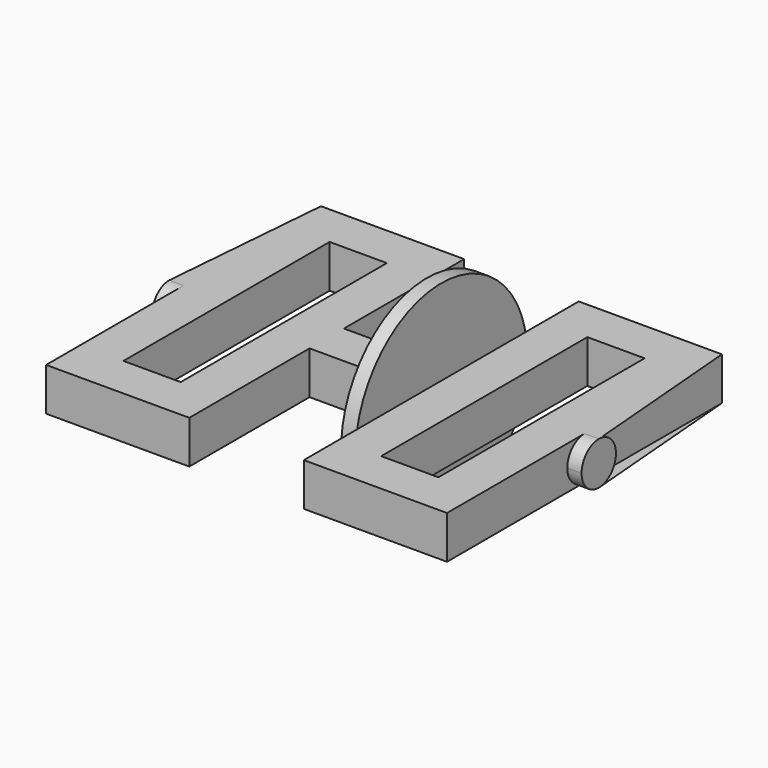
from build123d import *

# Parameters (mm, degrees)
F0_W     = 10
F0_H     = 30
F0_W_2   = 40
F0_H_2   = 180
F0_W_3   = 80
F1_DEPTH = 15
F2_R     = 15
F3_R     = 14.99999
F5_START = 30
F4_R     = 75
F5_DEPTH = 10


# Not quite as in the source:
# - a fillet or chamfer is up to 0.001 mm smaller than in the source, because OpenCascade refuses the exact size


with BuildPart() as f1:
    # F0 (on Top) → F1 (new body, symmetric)
    with BuildSketch(Plane.XY):
        with Locations((-145, 0)):
            Rectangle(F0_W, F0_H)
        Polygon((-140, 120), (-140, 15), (-140, -15), (-140, -120), (-40, -120), (-40, -15), (-40, 15), (-40, 120), align=None)
        with Locations((-90, 0)):
            Rectangle(F0_W_2, F0_H_2, mode=Mode.SUBTRACT)
        Rectangle(F0_W_3, F0_H)
        Polygon((40, 120), (40, 15), (40, -15), (40, -120), (140, -120), (140, -15), (140, 15), (140, 120), align=None)
        with Locations((90, 0)):
            Rectangle(F0_W_2, F0_H_2, mode=Mode.SUBTRACT)
        with Locations((145, 0)):
            Rectangle(F0_W, F0_H)
    extrude(amount=F1_DEPTH, both=True)

    # F2
    f2_edges = [f1.edges().sort_by_distance(p)[0] for p in [
        (-145, -15, 15),
    ]]
    fillet(f2_edges, radius=F2_R)

    # F3 (radius 15 in the source; OpenCascade refuses exactly that, so slightly less here)
    f3_edges = [f1.edges().sort_by_distance(p)[0] for p in [
        (-145, -15, -15),
        (-145, 15, -15),
        (-145, 15, 15),
        (145, 15, -15),
        (145, 15, 15),
        (145, -15, 15),
        (145, -15, -15),
    ]]
    fillet(f3_edges, radius=F3_R)


with BuildPart() as f5:
    # F4 (on Right) → F5 (new body)
    with BuildSketch(Plane.YZ.offset(F5_START)):
        Circle(F4_R)
    extrude(amount=F5_DEPTH)


solid = Compound([f1.part, f5.part])
